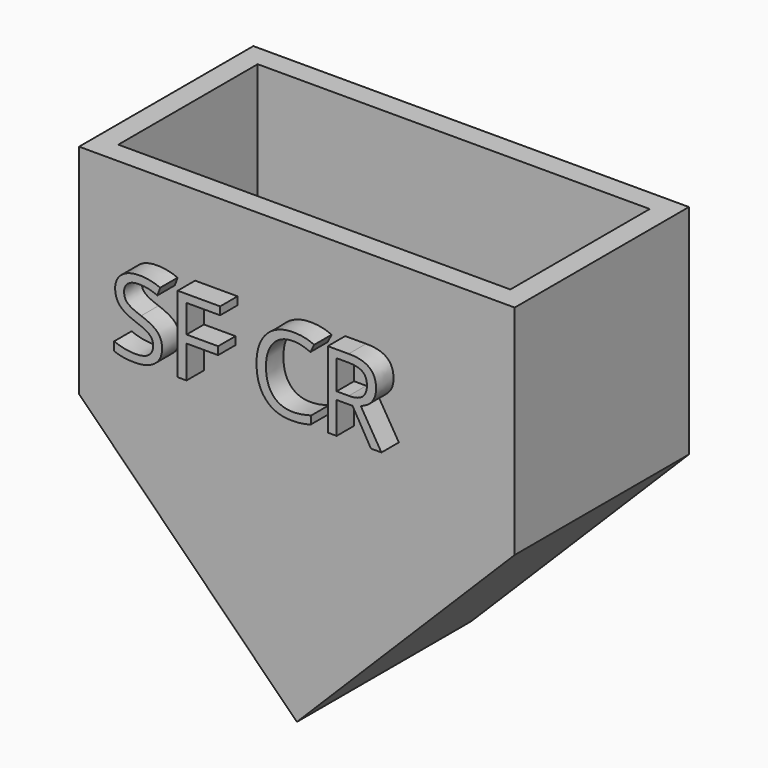
from build123d import *

# Parameters (mm, degrees)
F1_DEPTH     = 25.4
F2_T         = -2.54
F3_TEXT_SIZE = 12.4419628169
F4_DEPTH     = 2.54


# Not quite as in the source:
# - Text() gives the source's letters only with a copy of the font that has no kerning and outlines rounded to 1/6400 em; it was checked with that copy


with BuildPart() as f1:
    # F0 (on Front) → F1 (new body)
    with BuildSketch(Plane.XZ):
        Polygon((0, -25.4), (25.4, 0), (25.4, 25.4), (-25.4, 25.4), (-25.4, 0), align=None)
    extrude(amount=F1_DEPTH)

    # F2
    f2_openings = [f1.faces().sort_by_distance(p)[0] for p in [
        (0, -12.7, 25.4),
    ]]
    offset(amount=F2_T, openings=f2_openings)

    # F3 (on face) → F4 (join)
    with BuildSketch(Plane.XZ.offset(25.4)):
        with Locations((-19.919327204, 7.1633209368)):
            Text('SF CR', F3_TEXT_SIZE, font='Open Sans', text_align=(TextAlign.LEFT, TextAlign.BOTTOM))
    extrude(amount=F4_DEPTH)


solid = f1.part
